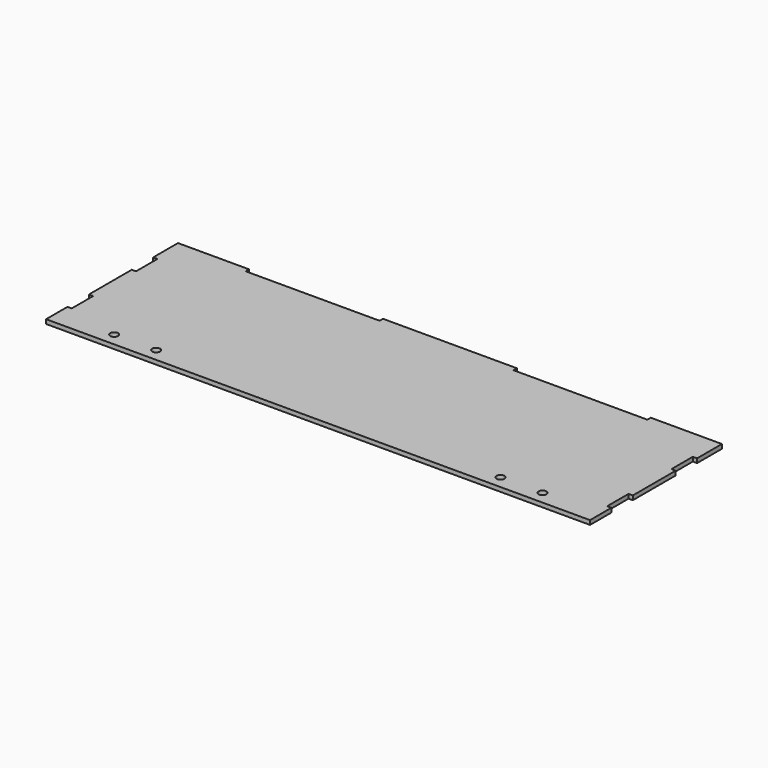
from build123d import *

# Parameters (mm, degrees)
F0_W     = 1.5875
F0_H     = 20
F0_H_2   = 10
F0_W_2   = 50
F0_H_3   = 1.5875
F0_W_3   = 200
F0_R     = 1.4732
F1_DEPTH = 1.5875


# Not quite as in the source:
# - a length typed as a fraction of an inch, garbled in the dataset ("3 / 203.2 mm" for 3/8 in), is restored


with BuildPart() as f1:
    # F0 (on Top) → F1 (new body)
    with BuildSketch(Plane.XY):
        with Locations((100.8545614919, -1.1143145161)):
            Rectangle(F0_W, F0_H)
        with Locations((-100.7329385081, -1.1143145161)):
            Rectangle(F0_W, F0_H)
        with Locations((-100.7329385081, -26.1143145161)):
            Rectangle(F0_W, F0_H_2)
        with Locations((100.8545614919, 23.8856854839)):
            Rectangle(F0_W, F0_H_2)
        with Locations((-100.7329385081, 23.8856854839)):
            Rectangle(F0_W, F0_H_2)
        with Locations((100.8545614919, -26.1143145161)):
            Rectangle(F0_W, F0_H_2)
        Polygon((75.0608114919, 28.8856854839), (100.0608114919, 28.8856854839), (101.6483114919, 28.8856854839), (101.6483114919, 30.4731854839), (75.0608114919, 30.4731854839), align=None)
        with Locations((0.0608114919, 29.6794354839)):
            Rectangle(F0_W_2, F0_H_3)
        Polygon((-101.5266885081, 28.8856854839), (-99.9391885081, 28.8856854839), (-74.9391885081, 28.8856854839), (-74.9391885081, 30.4731854839), (-101.5266885081, 30.4731854839), align=None)
        Polygon((100.0608114919, 8.8856854839), (100.0608114919, 18.8856854839), (-99.9391885081, 18.8856854839), (-99.9391885081, 8.8856854839), (-99.9391885081, -11.1143145161), (-99.9391885081, -21.1143145161), (100.0608114919, -21.1143145161), (100.0608114919, -11.1143145161), align=None)
        with Locations((0.0608114919, -26.1143145161)):
            Rectangle(F0_W_3, F0_H_2)
        with Locations((-79.9391885081, -26.3018145161)):
            Circle(F0_R, mode=Mode.SUBTRACT)
        with Locations((-64.2419885081, -26.3018145161)):
            Circle(F0_R, mode=Mode.SUBTRACT)
        with Locations((64.3636114919, -26.3018145161)):
            Circle(F0_R, mode=Mode.SUBTRACT)
        with Locations((80.0608114919, -26.3018145161)):
            Circle(F0_R, mode=Mode.SUBTRACT)
        Polygon((-99.9391885081, 18.8856854839), (100.0608114919, 18.8856854839), (100.0608114919, 28.8856854839), (75.0608114919, 28.8856854839), (25.0608114919, 28.8856854839), (-24.9391885081, 28.8856854839), (-74.9391885081, 28.8856854839), (-99.9391885081, 28.8856854839), align=None)
    extrude(amount=F1_DEPTH)


solid = f1.part
